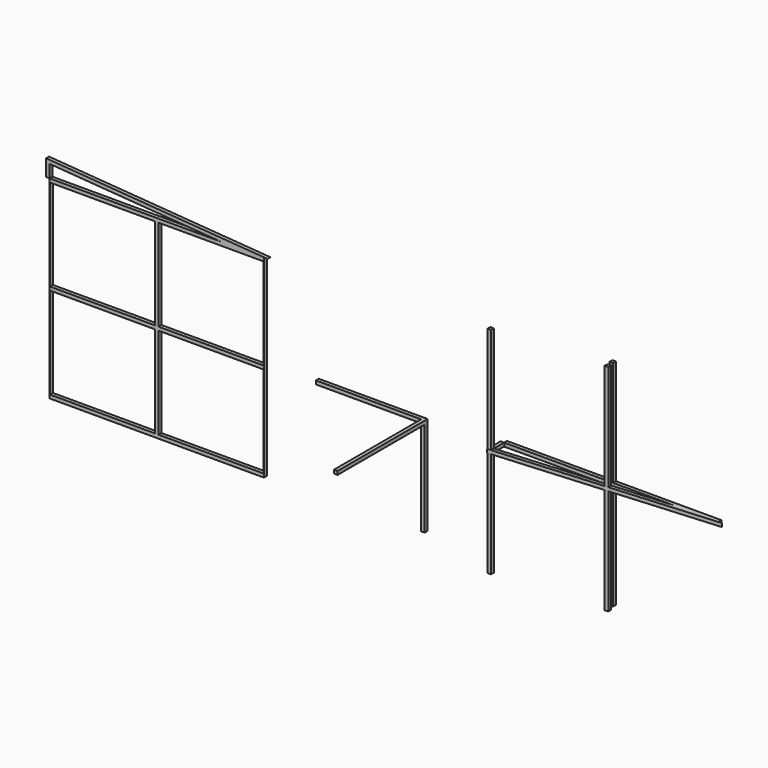
from build123d import *

# Parameters (mm, degrees)
F0_W     = 952
F0_H     = 32
F1_DEPTH = 33
F0_W_2   = 32
F0_H_2   = 952
F0_W_3   = 947.5
F0_H_3   = 827
F0_W_4   = 950.5
F2_W     = 32
F2_H     = 32
F3_DEPTH = 984
F5_DEPTH = 32
F6_W     = 32
F6_H     = 32
F7_DEPTH = 956
F8_DEPTH = 988


# Not quite as in the source:
# - a feature names something its author has since deleted; it is built from what else it names


with BuildPart() as f1:
    # F0 (on Front) → F1 (new body)
    with BuildSketch(Plane.XZ):
        Polygon((3356.2954444885, 34.6195969582), (3388.2954444885, 34.6195969582), (3388.2954444885, 925.6195969582), (3356.2954444885, 925.6195969582), (3356.2954444885, 893.6195969582), align=None)
        with Locations((2880.2954444885, 909.6195969582)):
            Rectangle(F0_W, F0_H)
    extrude(amount=F1_DEPTH)

    # F2 (on face) → F3 (join)
    with BuildSketch(Plane.XZ.offset(33)):
        with Locations((3372.2954444885, 909.6195969582)):
            Rectangle(F2_W, F2_H)
    extrude(amount=F3_DEPTH)


with BuildPart() as f1b:
    # F0 (on Front) → F1, piece 2 (new body)
    with BuildSketch(Plane.XZ):
        with Locations((5073.074546814, 1460)):
            Rectangle(F0_W_2, F0_H_2)
        with Locations((5073.074546814, 476)):
            Rectangle(F0_W_2, F0_H_2)
        with Locations((4581.074546814, 968)):
            Rectangle(F0_W, F0_H)
        with Locations((5565.074546814, 968)):
            Rectangle(F0_W, F0_H)
        with Locations((5073.074546814, 968)):
            Rectangle(F0_W_2, F0_H)
    extrude(amount=F1_DEPTH)

    # F4 (on face) → F5 (join)
    with BuildSketch(Plane(origin=(0, 0, 952), x_dir=(1, 0, 0), z_dir=(0, 0, -1))):
        Polygon((4073.074546814, 33), (4105.074546814, 33), (4107.3265075684, 33), (4107.3265075684, 35.0165888667), (4105.074546814, 35.0165888667), (4105.074546814, 148.5101262078), (5645.2095629178, 33), (6041.074546814, 33), (6073.074546814, 33), (4073.074546814, 183), align=None)
    extrude(amount=-F5_DEPTH)

    # F6 (on face) → F7 (join)
    with BuildSketch(Plane(origin=(0, 0, 952), x_dir=(1, 0, 0), z_dir=(0, 0, -1))):
        with Locations((4089.074546814, 164.5101262078)):
            Rectangle(F6_W, F6_H)
        Polygon((5073.3726069148, 107.8877717002), (5073.3726069148, 75.8877717002), (5105.2829848312, 73.4944933565), (5105.2829848312, 105.4944933565), align=None)
    extrude(amount=F7_DEPTH)

    # F6 (on face) → F8 (join)
    with BuildSketch(Plane(origin=(0, 0, 952), x_dir=(1, 0, 0), z_dir=(0, 0, -1))):
        with Locations((4089.074546814, 164.5101262078)):
            Rectangle(F6_W, F6_H)
        Polygon((5073.3726069148, 107.8877717002), (5073.3726069148, 75.8877717002), (5105.2829848312, 73.4944933565), (5105.2829848312, 105.4944933565), align=None)
    extrude(amount=-F8_DEPTH)


with BuildPart() as f1c:
    # F0 (on Front) → F1, piece 3 (new body)
    with BuildSketch(Plane.XZ):
        Polygon((0, 1750), (0, 0), (1933, 0), (1936, 0), (1936, 1750), (1968, 1750), (-32, 1900), (-32, 1750), align=None)
        with Locations((476.75, 445.5)):
            Rectangle(F0_W_3, F0_H_3, mode=Mode.SUBTRACT)
        with Locations((1457.75, 445.5)):
            Rectangle(F0_W_4, F0_H_3, mode=Mode.SUBTRACT)
        Polygon((982.5, 891), (982.5, 859), (950.5, 859), (950.5, 891), (3, 891), (3, 1718), (950.5, 1718), (982.5, 1718), (1933, 1718), (1933, 891), align=None, mode=Mode.SUBTRACT)
        Polygon((1540.1350161039, 1750), (1.2016075198, 1750), (1.2016075198, 1750.8734464645), (0, 1750.8734464645), (0, 1865.5101262078), align=None, mode=Mode.SUBTRACT)
        with Locations((966.5, 875)):
            Rectangle(F0_W_2, F0_H)
        with Locations((966.5, 1304.5)):
            Rectangle(F0_W_2, F0_H_3)
    extrude(amount=F1_DEPTH)


solid = Compound([f1.part, f1b.part, f1c.part])
